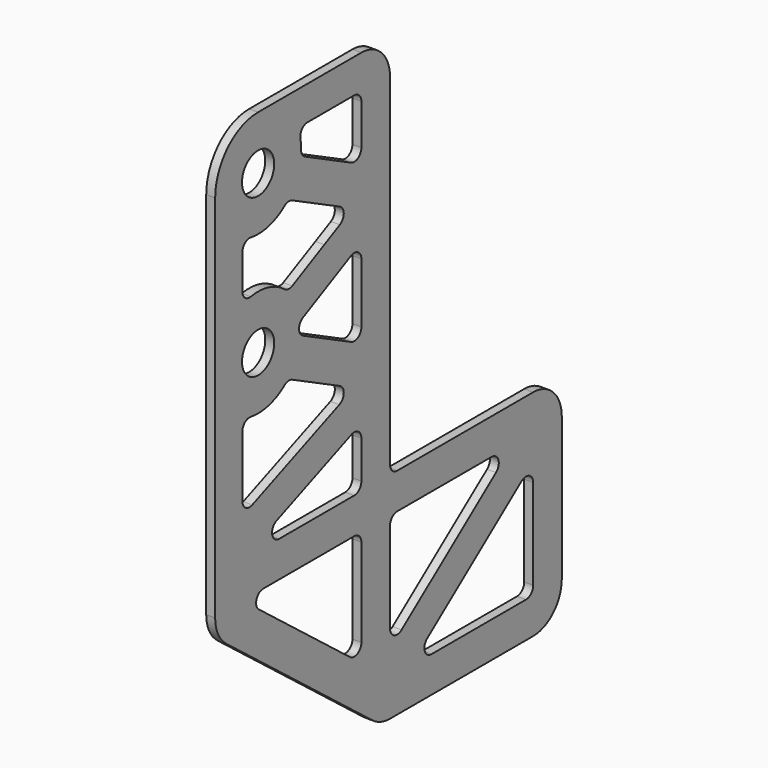
from build123d import *

# Parameters (mm, degrees)
F0_R     = 6.985
F1_DEPTH = 3.175
F3_D     = 14.2748


with BuildPart() as f1:
    # F0 (on Right) → F1 (new body)
    with BuildSketch(Plane.YZ):
        with BuildLine():
            ThreePointArc((38.1, -53.975), (34.3802561211, -44.9947438789), (25.4, -41.275))
            Line((25.4, -41.275), (-34.925, -41.275))
            ThreePointArc((-34.925, -41.275), (-37.1700640303, -40.3450640303), (-38.1, -38.1))
            Line((-38.1, -38.1), (-38.1, 41.275))
            Line((-38.1, 41.275), (-38.1, 47.5751108035))
            Line((-38.1, 47.5751108035), (-38.1, 83.1075017654))
            ThreePointArc((-38.1, 83.1075017654), (-41.8197438789, 92.0877578865), (-50.8, 95.8075017654))
            Line((-50.8, 95.8075017654), (-96.6180321919, 95.8075017654))
            ThreePointArc((-96.6180321919, 95.8075017654), (-110.0884163735, 90.227885947), (-115.6680321919, 76.7575017654))
            Line((-115.6680321919, 76.7575017654), (-115.6680321919, 19.1893243394))
            Line((-115.6680321919, 19.1893243394), (-115.6680321919, -54.4674657519))
            ThreePointArc((-115.6680321919, -54.4674657519), (-114.372733143, -60.0552019855), (-110.7510564099, -64.5031288602))
            Line((-110.7510564099, -64.5031288602), (-45.883024218, -114.8106631083))
            ThreePointArc((-45.883024218, -114.8106631083), (-42.2132151977, -116.7904675622), (-38.1, -117.475))
            Line((-38.1, -117.475), (25.4, -117.475))
            ThreePointArc((25.4, -117.475), (34.3802561211, -113.7552561211), (38.1, -104.775))
            Line((38.1, -104.775), (38.1, -53.975))
        make_face()
        with BuildLine():
            ThreePointArc((-50.8, -88.4454353572), (-52.5780659416, -91.2966105949), (-55.9207560545, -90.9543511342))
            Line((-55.9207560545, -90.9543511342), (-96.2740219927, -59.6589157771))
            ThreePointArc((-96.2740219927, -59.6589157771), (-97.3321328287, -56.1216962006), (-94.3282659382, -53.975))
            Line((-94.3282659382, -53.975), (-53.975, -53.975))
            ThreePointArc((-53.975, -53.975), (-51.7299359697, -54.9049359697), (-50.8, -57.15))
            Line((-50.8, -57.15), (-50.8, -88.4454353572))
        make_face(mode=Mode.SUBTRACT)
        with BuildLine():
            Line((-88.4453191039, -35.1558561059), (-55.1635460576, -21.7200589551))
            ThreePointArc((-55.1635460576, -21.7200589551), (-52.1991915549, -22.0322588212), (-50.8, -24.6642028492))
            Line((-50.8, -24.6642028492), (-50.8, -38.1))
            ThreePointArc((-50.8, -38.1), (-51.7299359697, -40.3450640303), (-53.975, -41.275))
            Line((-53.975, -41.275), (-87.2567730463, -41.275))
            ThreePointArc((-87.2567730463, -41.275), (-90.3735247098, -38.7053792763), (-88.4453191039, -35.1558561059))
        make_face(mode=Mode.SUBTRACT)
        with BuildLine():
            ThreePointArc((-38.1, -57.15), (-37.1700640303, -54.9049359697), (-34.925, -53.975))
            Line((-34.925, -53.975), (6.9827090181, -53.975))
            ThreePointArc((6.9827090181, -53.975), (9.9894060531, -56.1300010097), (8.9145691376, -59.6696312188))
            Line((8.9145691376, -59.6696312188), (-32.9931398805, -91.8012507785))
            ThreePointArc((-32.9931398805, -91.8012507785), (-36.3298076595, -92.1289236249), (-38.1, -89.2816195597))
            Line((-38.1, -89.2816195597), (-38.1, -57.15))
        make_face(mode=Mode.SUBTRACT)
        with BuildLine():
            Line((22.225, -104.775), (-19.6827090181, -104.775))
            ThreePointArc((-19.6827090181, -104.775), (-22.6894060531, -102.6199989903), (-21.6145691376, -99.0803687812))
            Line((-21.6145691376, -99.0803687812), (20.2931398805, -66.9487492215))
            ThreePointArc((20.2931398805, -66.9487492215), (23.6298076595, -66.6210763751), (25.4, -69.4683804403))
            Line((25.4, -69.4683804403), (25.4, -101.6))
            ThreePointArc((25.4, -101.6), (24.4700640303, -103.8450640303), (22.225, -104.775))
        make_face(mode=Mode.SUBTRACT)
        with BuildLine():
            ThreePointArc((-84.8587723654, 5.7476975385), (-83.2201096499, 6.408506351), (-81.481969716, 6.0910896656))
            Line((-81.481969716, 6.0910896656), (-60.3749057725, -4.4348041313))
            ThreePointArc((-60.3749057725, -4.4348041313), (-58.6193026557, -7.4013325865), (-60.6032857265, -10.2202409842))
            Line((-60.6032857265, -10.2202409842), (-99.2394861343, -25.8176116721))
            ThreePointArc((-99.2394861343, -25.8176116721), (-102.203840637, -25.505411806), (-103.6030321919, -22.8734677781))
            Line((-103.6030321919, -22.8734677781), (-103.6030321919, -1.1608908265))
            ThreePointArc((-103.6030321919, -1.1608908265), (-102.4716219082, 1.2689993092), (-99.8837464776, 1.9671082242))
            ThreePointArc((-99.8837464776, 1.9671082242), (-91.969560093, 2.2609528282), (-84.8587723654, 5.7476975385))
        make_face(mode=Mode.SUBTRACT)
        with BuildLine():
            ThreePointArc((-96.8477962041, 27.7163225865), (-91.7608044139, 25.7548199819), (-89.6330321919, 20.7351025284))
            ThreePointArc((-89.6330321919, 20.7351025284), (-91.7608044139, 15.715385075), (-96.8477962041, 13.7538824704))
            ThreePointArc((-96.8477962041, 13.7538824704), (-103.6030321919, 20.7351025284), (-96.8477962041, 27.7163225865))
        make_face(mode=Mode.SUBTRACT)
        with BuildLine():
            Line((-50.8, 31.3570788484), (-50.8, 10.1131262084))
            ThreePointArc((-50.8, 10.1131262084), (-52.304388598, 7.4131849973), (-55.3919260116, 7.2718332496))
            Line((-55.3919260116, 7.2718332496), (-76.6916595751, 17.8938095697))
            ThreePointArc((-76.6916595751, 17.8938095696), (-78.4497335635, 20.7351025284), (-76.6916595751, 23.5763954872))
            Line((-76.6916595751, 23.5763954872), (-61.5697646385, 31.117541927))
            Line((-61.5697646385, 31.117541927), (-55.3919260116, 34.1983718072))
            ThreePointArc((-55.3919260116, 34.1983718072), (-52.304388598, 34.0570200595), (-50.8, 31.3570788484))
        make_face(mode=Mode.SUBTRACT)
        with BuildLine():
            Line((-67.2374686849, 42.4827137621), (-81.481969716, 35.3791153912))
            ThreePointArc((-81.481969716, 35.3791153912), (-83.2201096499, 35.0616987058), (-84.8587723654, 35.7225075184))
            ThreePointArc((-84.8587723654, 35.7225075184), (-91.969560093, 39.2092522286), (-99.8837464776, 39.5030968327))
            ThreePointArc((-99.8837464776, 39.5030968327), (-102.4716219082, 40.2012057477), (-103.6030321919, 42.6310958834))
            Line((-103.6030321919, 42.6310958834), (-103.6030321919, 54.8615084105))
            ThreePointArc((-103.6030321919, 54.8615084105), (-102.4716219082, 57.2913985461), (-99.8837464776, 57.9895074612))
            ThreePointArc((-99.8837464776, 57.9895074612), (-91.969560093, 58.2833520652), (-84.8587723653, 61.7700967755))
            ThreePointArc((-84.8587723654, 61.7700967755), (-83.2201096499, 62.430905588), (-81.481969716, 62.1134889026))
            Line((-81.481969716, 62.1134889026), (-60.3749057725, 51.5875951057))
            ThreePointArc((-60.3749057725, 51.5875951057), (-58.6168317841, 48.7463021469), (-60.3749057725, 45.9050091881))
            Line((-60.3749057725, 45.9050091882), (-67.2374686849, 42.4827137621))
        make_face(mode=Mode.SUBTRACT)
        with Locations((-96.6180321919, 76.7575017654)):
            Circle(F0_R, mode=Mode.SUBTRACT)
        with BuildLine():
            Line((-55.3919260116, 63.2942324866), (-75.8142656696, 73.4786607378))
            ThreePointArc((-75.8142656696, 73.4786607378), (-77.1135956749, 74.6760016746), (-77.5717243057, 76.3824605635))
            ThreePointArc((-77.5717243057, 76.3824605635), (-77.6234503942, 78.209521852), (-77.8500378876, 80.0232160511))
            ThreePointArc((-77.8500378876, 80.0232160511), (-77.1519289726, 82.6110914817), (-74.7220388369, 83.7425017654))
            Line((-74.7220388369, 83.7425017654), (-53.975, 83.7425017654))
            ThreePointArc((-53.975, 83.7425017654), (-51.7299359697, 82.8125657957), (-50.8, 80.5675017654))
            Line((-50.8, 80.5675017654), (-50.8, 66.1355254454))
            ThreePointArc((-50.8, 66.1355254454), (-52.304388598, 63.4355842343), (-55.3919260116, 63.2942324866))
        make_face(mode=Mode.SUBTRACT)
        with Locations((-96.6180321919, 76.7575017654)):
            Circle(F0_R)
    extrude(amount=F1_DEPTH)

    # F3 (through all)
    with Locations(Plane(origin=(0, 0, 0), x_dir=(0, -1, 0), z_dir=(-1, 0, 0))):
        with Locations((96.6180321919, 20.7351025284), (96.6180321919, 76.7575017654)):
            Hole(F3_D / 2)


solid = f1.part
